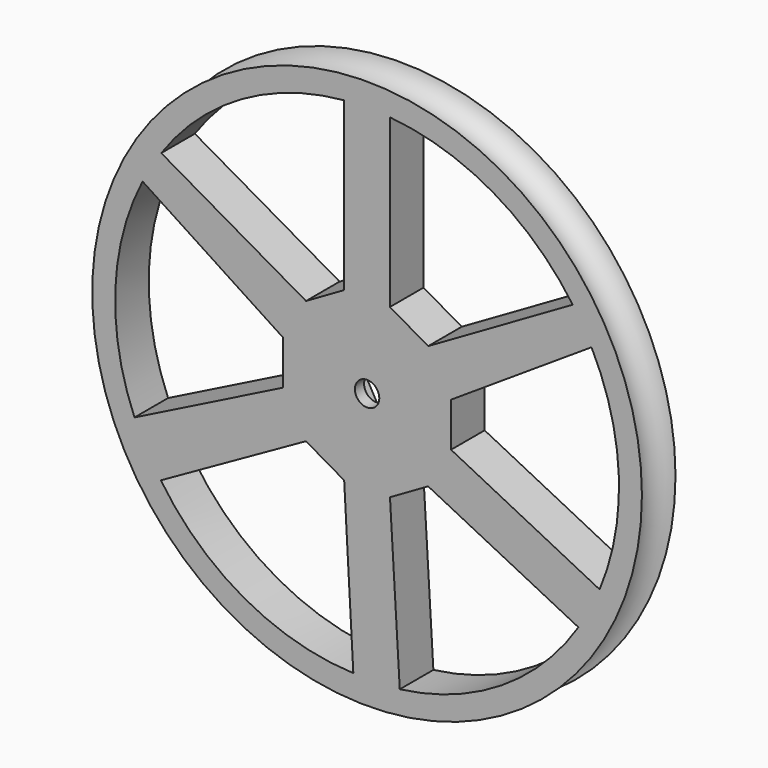
from build123d import *

# Parameters (mm, degrees)
F2_R     = 2.032
F3_DEPTH = 15.875
F4_DEPTH = 10.2362


# Not quite as in the source:
# - a feature names something its author has since deleted; it is built from what else it names


with BuildPart() as f1:
    # F0 (on Top) → F1 (revolve)
    with BuildSketch(Plane.XY):
        with BuildLine():
            Line((0, -5.1666409709), (0, -12.1516409709))
            Line((0, -12.1516409709), (45.72, -12.1516409709))
            ThreePointArc((45.72, -12.1516409709), (42.9147529825, -8.6591409709), (45.72, -5.1666409709))
            Line((45.72, -5.1666409709), (0, -5.1666409709))
        make_face()
    revolve(axis=Axis((0, -8.561744864, 0), (0, 1, 0)))

    # F2 (on Front) → F3 (cut)
    with BuildSketch(Plane.XZ):
        with BuildLine():
            Line((13.97, 3.6661742094), (13.97, -3.6661742094))
            Line((13.97, -3.6661742094), (38.6802071591, -16.0932599922))
            ThreePointArc((38.6802071591, -16.0932599922), (41.8782799617, 1.5705660984), (37.3345500424, 18.9369975174))
            Line((37.3345500424, 18.9369975174), (13.97, 3.6661742094))
        make_face()
        with BuildLine():
            Line((3.81, 41.7094333604), (3.81, 13.9314619955))
            Line((3.81, 13.9314619955), (10.16, 10.2652877862))
            Line((10.16, 10.2652877862), (34.2119266748, 24.1516741264))
            ThreePointArc((34.2119266748, 24.1516741264), (20.9542761873, 36.2954737188), (3.81, 41.7094333604))
        make_face()
        with BuildLine():
            Line((-34.2388233597, 24.0958361272), (-10.16, 10.2652877862))
            Line((-10.16, 10.2652877862), (-3.81, 13.9314619955))
            Line((-3.81, 13.9314619955), (-3.81, 41.7173788368))
            ThreePointArc((-3.81, 41.7173788368), (-20.9781685322, 36.2803485402), (-34.2388233597, 24.0958361272))
        make_face()
        with BuildLine():
            Line((-38.6893950171, -16.0623838358), (-13.97, -3.6661742094))
            Line((-13.97, -3.6661742094), (-13.97, 3.6661742094))
            Line((-13.97, 3.6661742094), (-37.3405062231, 18.9372899969))
            ThreePointArc((-37.3405062231, 18.9372899969), (-41.8787701809, 1.5863648371), (-38.6893950171, -16.0623838358))
        make_face()
        with BuildLine():
            Line((-3.81, -13.9314619955), (-10.16, -10.2652877862))
            Line((-10.16, -10.2652877862), (-34.3038742814, -23.844345572))
            ThreePointArc((-34.3038742814, -23.844345572), (-20.4303998238, -36.5921428083), (-2.2874128339, -41.6726596109))
            Line((-2.2874128339, -41.6726596109), (-3.81, -13.9314619955))
        make_face()
        with BuildLine():
            Line((10.16, -10.2652877862), (3.81, -13.9314619955))
            Line((3.81, -13.9314619955), (5.4400267393, -41.5192010913))
            ThreePointArc((5.4400267393, -41.5192010913), (22.3730839146, -35.4381883413), (35.1536490306, -22.7746857971))
            Line((35.1536490306, -22.7746857971), (10.16, -10.2652877862))
        make_face()
        Circle(F2_R)
    extrude(amount=F3_DEPTH, mode=Mode.SUBTRACT)

    # F2 (on Front) → F4 (cut)
    with BuildSketch(Plane.XZ):
        Polygon((-7.0386894402, 0.071686571), (-3.5814271117, -6.059840579), (3.4572623285, -6.1315271501), (7.0386894402, -0.071686571), (3.5814271117, 6.059840579), (-3.4572623285, 6.1315271501), align=None)
        Circle(F2_R, mode=Mode.SUBTRACT)
    extrude(amount=F4_DEPTH, mode=Mode.SUBTRACT)


solid = f1.part
